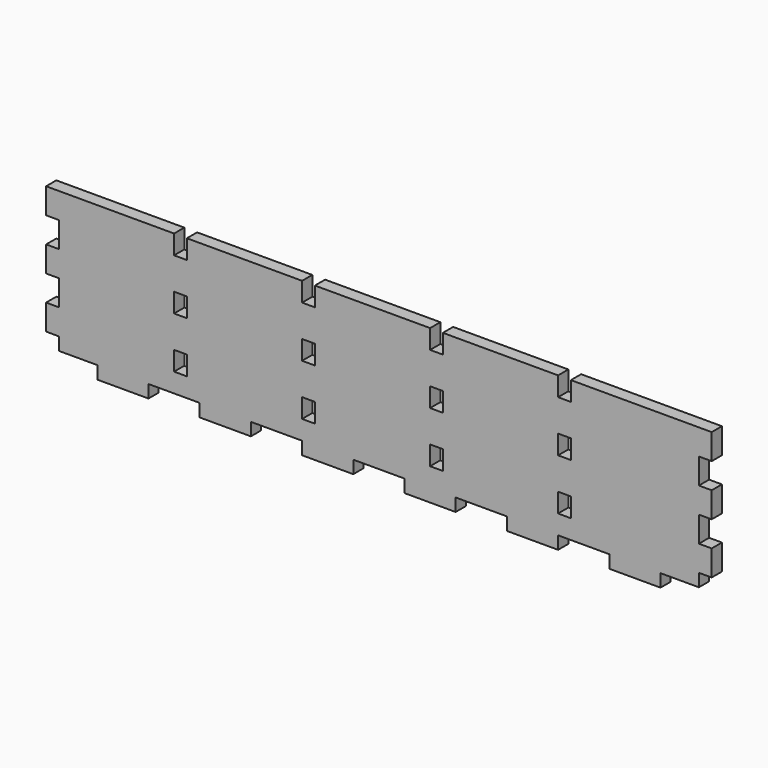
from build123d import *

# Parameters (mm, degrees)
F0_W     = 330.2
F0_H     = 76.2
F1_DEPTH = 6.35
F2_W     = 25.4
F2_H     = 6.35
F2_W_2   = 6.35
F2_H_2   = 12.7
F3_DEPTH = 6.35
F4_W     = 6.35
F4_H     = 9.525
F5_DEPTH = 6.35
F6_W     = 6.35
F6_H     = 6.35
F7_DEPTH = 6.35


# Not quite as in the source:
# - a feature names something its author has since deleted; it is built from what else it names


with BuildPart() as f1:
    # F0 (on Front) → F1 (new body)
    with BuildSketch(Plane.XZ):
        Rectangle(F0_W, F0_H)
    extrude(amount=F1_DEPTH)

    # F2 (on face) → F3 (cut, through all)
    with BuildSketch(Plane.XZ.offset(6.35)):
        with Locations((-152.4, -34.925)):
            Rectangle(F2_W, F2_H)
        with Locations((-101.6, -34.925)):
            Rectangle(F2_W, F2_H)
        with Locations((-50.8, -34.925)):
            Rectangle(F2_W, F2_H)
        with Locations((0, -34.925)):
            Rectangle(F2_W, F2_H)
        with Locations((50.8, -34.925)):
            Rectangle(F2_W, F2_H)
        with Locations((101.6, -34.925)):
            Rectangle(F2_W, F2_H)
        with Locations((152.4, -34.925)):
            Rectangle(F2_W, F2_H)
        with Locations((-161.925, -6.35)):
            Rectangle(F2_W_2, F2_H_2)
        with Locations((-161.925, 19.05)):
            Rectangle(F2_W_2, F2_H_2)
        with Locations((161.925, 19.05)):
            Rectangle(F2_W_2, F2_H_2)
        with Locations((161.925, -6.35)):
            Rectangle(F2_W_2, F2_H_2)
    extrude(amount=-F3_DEPTH, mode=Mode.SUBTRACT)

    # F4 (on face) → F5 (cut, through all)
    with BuildSketch(Plane.XZ.offset(6.35)):
        with Locations((-98.425, 33.3375)):
            Rectangle(F4_W, F4_H)
        with Locations((-98.425, 7.9375)):
            Rectangle(F4_W, F4_H)
        with Locations((-98.425, -17.4625)):
            Rectangle(F4_W, F4_H)
        with Locations((-34.925, 7.9375)):
            Rectangle(F4_W, F4_H)
        with Locations((-34.925, 33.3375)):
            Rectangle(F4_W, F4_H)
        with Locations((-34.925, -17.4625)):
            Rectangle(F4_W, F4_H)
        with Locations((28.575, 7.9375)):
            Rectangle(F4_W, F4_H)
        with Locations((28.575, 33.3375)):
            Rectangle(F4_W, F4_H)
        with Locations((28.575, -17.4625)):
            Rectangle(F4_W, F4_H)
        with Locations((92.075, -17.4625)):
            Rectangle(F4_W, F4_H)
        with Locations((92.075, 7.9375)):
            Rectangle(F4_W, F4_H)
        with Locations((92.075, 33.3375)):
            Rectangle(F4_W, F4_H)
    extrude(amount=-F5_DEPTH, mode=Mode.SUBTRACT)

    # F6 (on face) → F7 (cut, through all)
    with BuildSketch(Plane.XZ.offset(6.35)):
        with Locations((-161.925, -28.575)):
            Rectangle(F6_W, F6_H)
        with Locations((161.925, -28.575)):
            Rectangle(F6_W, F6_H)
    extrude(amount=-F7_DEPTH, mode=Mode.SUBTRACT)


solid = f1.part
